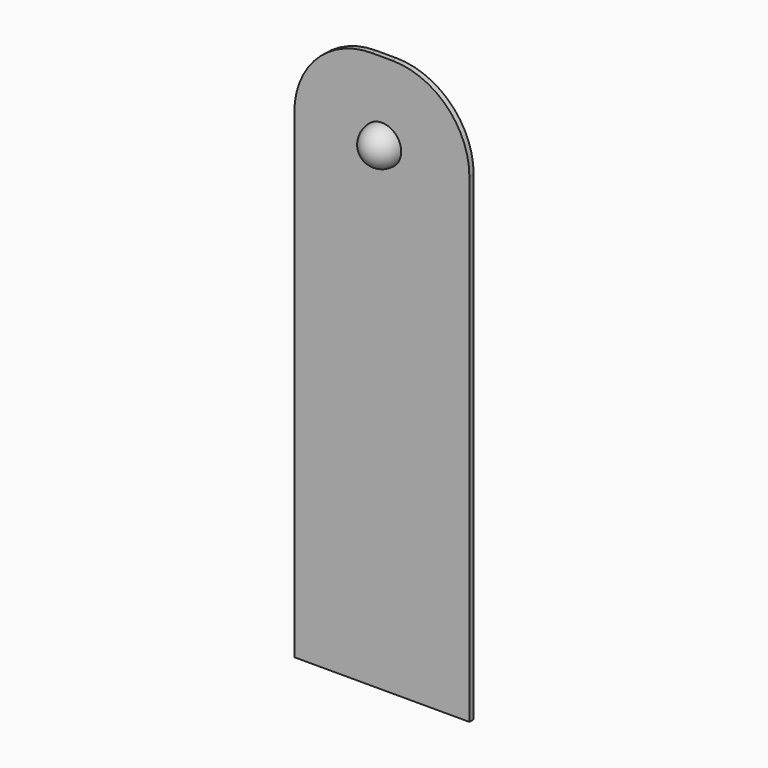
from build123d import *

# Parameters (mm, degrees)
F0_W     = 574.675
F0_H     = 1828.8
F1_DEPTH = 17.4625
F2_R     = 254
F3_R     = 254
F4_R     = 63.5
F5_DEPTH = 63.5
F6_R     = 63.49999


# Not quite as in the source:
# - a fillet or chamfer is up to 0.001 mm smaller than in the source, because OpenCascade refuses the exact size


with BuildPart() as f1:
    # F0 (on Front) → F1 (new body)
    with BuildSketch(Plane.XZ):
        with Locations((-1034.1491804612, -4.0362142026)):
            Rectangle(F0_W, F0_H)
    extrude(amount=F1_DEPTH)

    # F2
    f2_edges = [f1.edges().sort_by_distance(p)[0] for p in [
        (-1321.48668, -8.73125, 910.363786),
    ]]
    fillet(f2_edges, radius=F2_R)

    # F3
    f3_edges = [f1.edges().sort_by_distance(p)[0] for p in [
        (-746.81168, -8.73125, 910.363786),
    ]]
    fillet(f3_edges, radius=F3_R)

    # F4 (on face) → F5 (join)
    with BuildSketch(Plane.XZ.offset(17.4625)):
        with Locations((-1034.1491804612, 656.3637857974)):
            Circle(F4_R)
    extrude(amount=F5_DEPTH)

    # F6 (radius 63.5 in the source; OpenCascade refuses exactly that, so slightly less here)
    f6_edges = [f1.edges().sort_by_distance(p)[0] for p in [
        (-1097.64918, -80.9625, 656.363786),
    ]]
    fillet(f6_edges, radius=F6_R)


solid = f1.part
